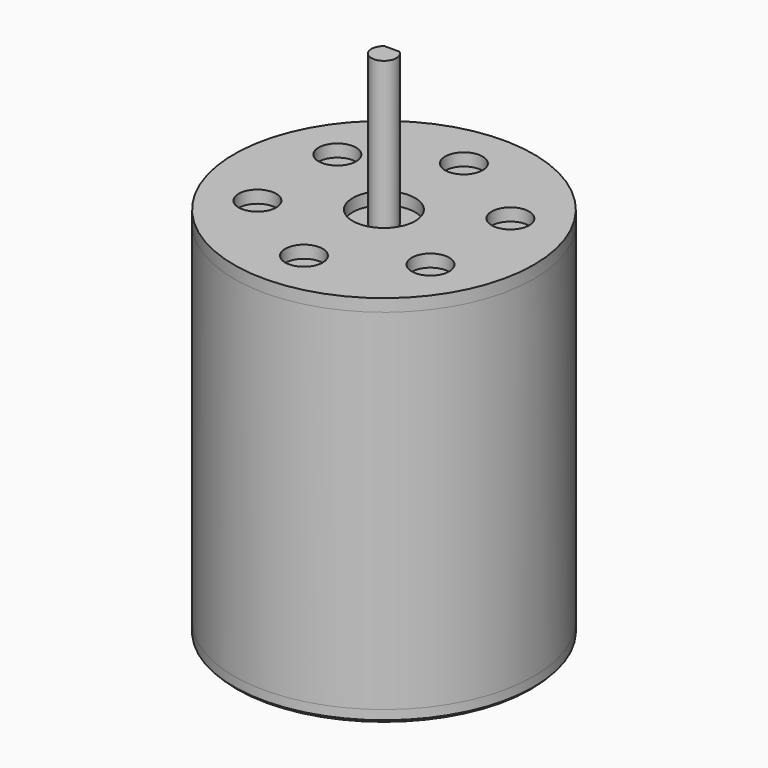
from build123d import *

# Parameters (mm, degrees)
F2_R     = 12
F2_R_2   = 1.5
F2_R_3   = 2.5
F3_DEPTH = 1
F4_START = 1
F4_DEPTH = 28
F5_START = 29
F5_DEPTH = 1
F6_START = 29
F6_DEPTH = 12
F7_SIZE  = 0.25


with BuildPart() as f3:
    # F2 (on Top) → F3 (new body)
    with BuildSketch(Plane.XY):
        Circle(F2_R)
        with Locations((-6.9282032303, -4)):
            Circle(F2_R_2, mode=Mode.SUBTRACT)
        with Locations((0, -8)):
            Circle(F2_R_2, mode=Mode.SUBTRACT)
        with Locations((6.9282032303, -4)):
            Circle(F2_R_2, mode=Mode.SUBTRACT)
        with Locations((-6.9282032303, 4)):
            Circle(F2_R_2, mode=Mode.SUBTRACT)
        Circle(F2_R_3, mode=Mode.SUBTRACT)
        with Locations((6.9282032303, 4)):
            Circle(F2_R_2, mode=Mode.SUBTRACT)
        with Locations((0, 8)):
            Circle(F2_R_2, mode=Mode.SUBTRACT)
        with Locations((-6.9282032303, 4)):
            Circle(F2_R_2)
        with Locations((-6.9282032303, -4)):
            Circle(F2_R_2)
        with Locations((0, -8)):
            Circle(F2_R_2)
        with Locations((6.9282032303, -4)):
            Circle(F2_R_2)
        with Locations((6.9282032303, 4)):
            Circle(F2_R_2)
        with Locations((0, 8)):
            Circle(F2_R_2)
    extrude(amount=F3_DEPTH)

    # F7
    f7_edges = [f3.edges().sort_by_distance(p)[0] for p in [
        (-12, 0, 0),
    ]]
    chamfer(f7_edges, length=F7_SIZE)


with BuildPart() as f4:
    # F2 (on Top) → F4 (new body)
    with BuildSketch(Plane.XY.offset(F4_START)):
        Circle(F2_R)
        with Locations((-6.9282032303, -4)):
            Circle(F2_R_2, mode=Mode.SUBTRACT)
        with Locations((0, -8)):
            Circle(F2_R_2, mode=Mode.SUBTRACT)
        with Locations((6.9282032303, -4)):
            Circle(F2_R_2, mode=Mode.SUBTRACT)
        with Locations((-6.9282032303, 4)):
            Circle(F2_R_2, mode=Mode.SUBTRACT)
        Circle(F2_R_3, mode=Mode.SUBTRACT)
        with Locations((6.9282032303, 4)):
            Circle(F2_R_2, mode=Mode.SUBTRACT)
        with Locations((0, 8)):
            Circle(F2_R_2, mode=Mode.SUBTRACT)
        Circle(F2_R_3)
        with BuildLine():
            ThreePointArc((0.6, 0.8), (0.894427191, 0.4472135955), (1, 0))
            ThreePointArc((1, 0), (-0.4472135955, -0.894427191), (-0.6, 0.8))
            ThreePointArc((-0.6, 0.8), (0, 1), (0.6, 0.8))
        make_face(mode=Mode.SUBTRACT)
        with Locations((-6.9282032303, -4)):
            Circle(F2_R_2)
        with Locations((0, -8)):
            Circle(F2_R_2)
        with Locations((6.9282032303, 4)):
            Circle(F2_R_2)
        with Locations((6.9282032303, -4)):
            Circle(F2_R_2)
        with Locations((0, 8)):
            Circle(F2_R_2)
        with Locations((-6.9282032303, 4)):
            Circle(F2_R_2)
        with BuildLine():
            ThreePointArc((-0.6, 0.8), (-0.4472135955, -0.894427191), (1, 0))
            ThreePointArc((1, 0), (0.894427191, 0.4472135955), (0.6, 0.8))
            Line((0.6, 0.8), (-0.6, 0.8))
        make_face()
        with BuildLine():
            Line((-0.6, 0.8), (0.6, 0.8))
            ThreePointArc((0.6, 0.8), (0, 1), (-0.6, 0.8))
        make_face()
    extrude(amount=F4_DEPTH)


with BuildPart() as f5:
    # F2 (on Top) → F5 (new body)
    with BuildSketch(Plane.XY.offset(F5_START)):
        Circle(F2_R)
        with Locations((-6.9282032303, -4)):
            Circle(F2_R_2, mode=Mode.SUBTRACT)
        with Locations((0, -8)):
            Circle(F2_R_2, mode=Mode.SUBTRACT)
        with Locations((6.9282032303, -4)):
            Circle(F2_R_2, mode=Mode.SUBTRACT)
        with Locations((-6.9282032303, 4)):
            Circle(F2_R_2, mode=Mode.SUBTRACT)
        Circle(F2_R_3, mode=Mode.SUBTRACT)
        with Locations((6.9282032303, 4)):
            Circle(F2_R_2, mode=Mode.SUBTRACT)
        with Locations((0, 8)):
            Circle(F2_R_2, mode=Mode.SUBTRACT)
    extrude(amount=F5_DEPTH)


with BuildPart() as f6:
    # F2 (on Top) → F6 (new body)
    with BuildSketch(Plane.XY.offset(F6_START)):
        with BuildLine():
            ThreePointArc((-0.6, 0.8), (-0.4472135955, -0.894427191), (1, 0))
            ThreePointArc((1, 0), (0.894427191, 0.4472135955), (0.6, 0.8))
            Line((0.6, 0.8), (-0.6, 0.8))
        make_face()
    extrude(amount=F6_DEPTH)


solid = Compound([f3.part, f4.part, f5.part, f6.part])
